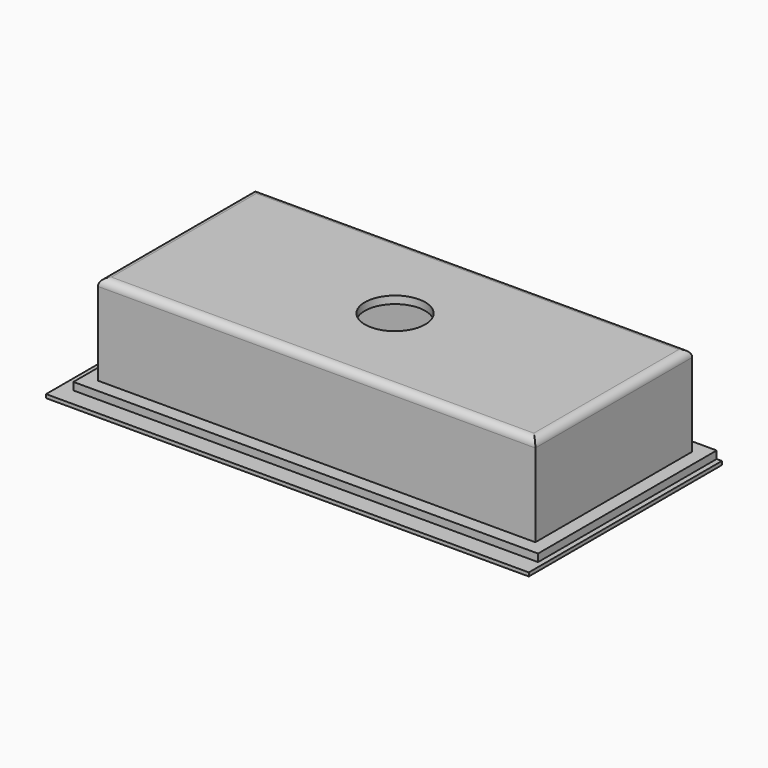
from build123d import *

# Parameters (mm, degrees)
F0_W      = 88.9
F0_H      = 38.1
F1_DEPTH  = 17.4625
F2_T      = 1.5875
F3_W      = 97.79
F3_H      = 46.99
F3_W_2    = 88.9
F3_H_2    = 38.1
F4_DEPTH  = 1.5875
F5_R      = 1.5875
F6_R      = 6.35
F7_DEPTH  = 25.4
F8_W      = 97.79
F8_H      = 46.99
F8_W_2    = 88.9
F8_H_2    = 38.1
F9_DEPTH  = 0.762
F10_R     = 4.445
F11_DEPTH = 0.762


with BuildPart() as f1:
    # F0 (on Top) → F1 (new body)
    with BuildSketch(Plane.XY):
        Rectangle(F0_W, F0_H)
    extrude(amount=F1_DEPTH)

    # F2
    f2_openings = [f1.faces().sort_by_distance(p)[0] for p in [
        (0, 0, 0),
    ]]
    offset(amount=F2_T, openings=f2_openings, kind=Kind.INTERSECTION)

    # F3 (on face) → F4 (join)
    with BuildSketch(Plane(origin=(0, 0, 0), x_dir=(1, 0, 0), z_dir=(0, 0, -1))):
        Rectangle(F3_W, F3_H)
        Rectangle(F3_W_2, F3_H_2, mode=Mode.SUBTRACT)
    extrude(amount=F4_DEPTH)

    # F5
    f5_edges = [f1.edges().sort_by_distance(p)[0] for p in [
        (46.0375, 0, 19.05),
        (0, -20.6375, 19.05),
        (-46.0375, 0, 19.05),
        (0, 20.6375, 19.05),
    ]]
    fillet(f5_edges, radius=F5_R)

    # F6 (on face) → F7 (cut)
    with BuildSketch(Plane.XY.offset(19.05)):
        Circle(F6_R)
    extrude(amount=-F7_DEPTH, mode=Mode.SUBTRACT)


with BuildPart() as f9:
    # F8 (on face) → F9 (new body)
    with BuildSketch(Plane(origin=(0, 0, -1.5875), x_dir=(1, 0, 0), z_dir=(0, 0, -1))):
        Polygon((49.9999, 27.305), (-51.6001, 27.305), (-51.6001, -23.495), (-48.895, -23.495), (-48.895, 23.495), (48.895, 23.495), (48.895, -23.495), (49.9999, -23.495), align=None)
        Rectangle(F8_W, F8_H)
        Rectangle(F8_W_2, F8_H_2, mode=Mode.SUBTRACT)
        Rectangle(F8_W_2, F8_H_2)
    extrude(amount=F9_DEPTH)

    # F10 (on face) → F11 (cut, through all)
    with BuildSketch(Plane.XY.offset(-1.5875)):
        Circle(F10_R)
    extrude(amount=-F11_DEPTH, mode=Mode.SUBTRACT)


solid = Compound([f1.part, f9.part])
